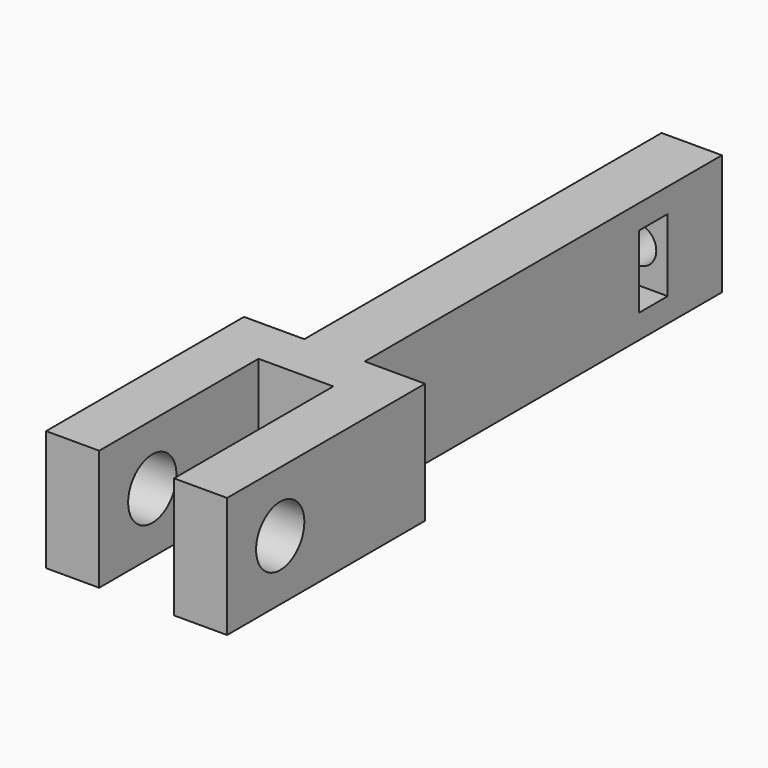
from build123d import *

# Parameters (mm, degrees)
F0_W          = 5
F0_H          = 10
F0_R          = 1.55
F1_DEPTH      = 37
F2_W          = 15
F2_H          = 10
F3_DEPTH      = 4
F4_W          = 4.4
F4_H          = 10
F5_DEPTH      = 16.5
F6_R          = 2.5
F7_DEPTH      = 4.401
F7_DEPTH_BACK = 10.601
F8_W          = 3
F8_H          = 6
F9_DEPTH      = 10.001


# Not quite as in the source:
# - a feature names something its author has since deleted; it is built from what else it names


with BuildPart() as f1:
    # F0 (on Front) → F1 (new body)
    with BuildSketch(Plane.XZ):
        Rectangle(F0_W, F0_H)
        Circle(F0_R, mode=Mode.SUBTRACT)
    extrude(amount=F1_DEPTH)

    # F2 (on face) → F3 (join)
    with BuildSketch(Plane.XZ.offset(37)):
        Rectangle(F2_W, F2_H)
    extrude(amount=F3_DEPTH)

    # F4 (on face) → F5 (join)
    with BuildSketch(Plane.XZ.offset(41)):
        with Locations((-5.3, 0)):
            Rectangle(F4_W, F4_H)
        with Locations((5.3, 0)):
            Rectangle(F4_W, F4_H)
    extrude(amount=F5_DEPTH)

    # F6 (on face) → F7 (cut, two sides)
    with BuildSketch(Plane.YZ.offset(-3.1)) as f7_sk:
        with Locations((-52, 0)):
            Circle(F6_R)
    extrude(amount=-F7_DEPTH, mode=Mode.SUBTRACT)
    extrude(f7_sk.sketch, amount=F7_DEPTH_BACK, mode=Mode.SUBTRACT)

    # F8 (on face) → F9 (cut, through all)
    with BuildSketch(Plane(origin=(-2.5, 0, 0), x_dir=(0, -1, 0), z_dir=(-1, 0, 0))):
        with Locations((7.1113700978, 0)):
            Rectangle(F8_W, F8_H)
    extrude(amount=-F9_DEPTH, mode=Mode.SUBTRACT)


solid = f1.part
